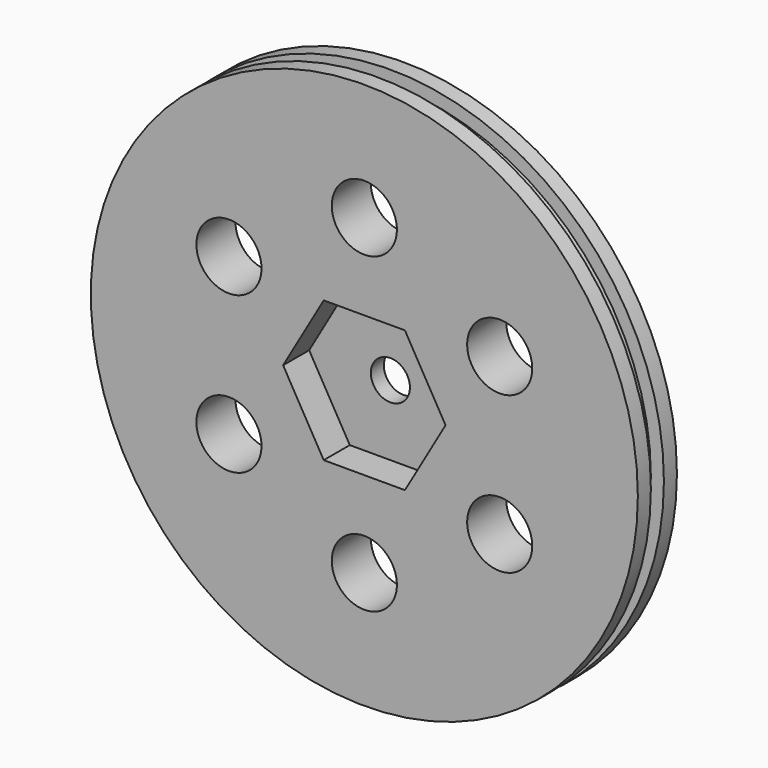
from build123d import *

# Parameters (mm, degrees)
F0_R     = 26.67
F0_R_2   = 25.4
F1_DEPTH = 1.5875
F2_R     = 25.4
F3_DEPTH = 1.5875
F4_R     = 26.67
F4_R_2   = 25.4
F5_DEPTH = 1.5875
F6_R     = 1.905
F7_DEPTH = 25.4
F9_D     = 6.35


# Not quite as in the source:
# - a length typed as a fraction of an inch, garbled in the dataset ("3 / 203.2 mm" for 3/8 in), is restored


with BuildPart() as f1:
    # F0 (on Front) → F1 (new body)
    with BuildSketch(Plane.XZ):
        Circle(F0_R)
        Circle(F0_R_2, mode=Mode.SUBTRACT)
        Circle(F0_R_2)
        with BuildLine():
            ThreePointArc((3.9594681461, 6.858), (6.858, 3.9594681461), (7.9189362922, 0))
            ThreePointArc((7.9189362922, 0), (6.858, -3.9594681461), (3.9594681461, -6.858))
            ThreePointArc((3.9594681461, -6.858), (0, -7.9189362922), (-3.9594681461, -6.858))
            ThreePointArc((-3.9594681461, -6.858), (-6.858, -3.9594681461), (-7.9189362922, 0))
            ThreePointArc((-7.9189362922, 0), (-6.858, 3.9594681461), (-3.9594681461, 6.858))
            ThreePointArc((-3.9594681461, 6.858), (0, 7.9189362922), (3.9594681461, 6.858))
        make_face(mode=Mode.SUBTRACT)
        Polygon((3.9594681461, -6.858), (7.9189362922, 0), (3.9594681461, 6.858), (-3.9594681461, 6.858), (-7.9189362922, 0), (-3.9594681461, -6.858), align=None)
        with BuildLine():
            Line((-3.9594681461, 6.858), (3.9594681461, 6.858))
            ThreePointArc((3.9594681461, 6.858), (0, 7.9189362922), (-3.9594681461, 6.858))
        make_face()
        with BuildLine():
            Line((3.9594681461, 6.858), (7.9189362922, 0))
            ThreePointArc((7.9189362922, 0), (6.858, 3.9594681461), (3.9594681461, 6.858))
        make_face()
        with BuildLine():
            ThreePointArc((3.9594681461, -6.858), (6.858, -3.9594681461), (7.9189362922, 0))
            Line((7.9189362922, 0), (3.9594681461, -6.858))
        make_face()
        with BuildLine():
            ThreePointArc((-3.9594681461, -6.858), (0, -7.9189362922), (3.9594681461, -6.858))
            Line((3.9594681461, -6.858), (-3.9594681461, -6.858))
        make_face()
        with BuildLine():
            ThreePointArc((-7.9189362922, 0), (-6.858, -3.9594681461), (-3.9594681461, -6.858))
            Line((-3.9594681461, -6.858), (-7.9189362922, 0))
        make_face()
        with BuildLine():
            Line((-7.9189362922, 0), (-3.9594681461, 6.858))
            ThreePointArc((-3.9594681461, 6.858), (-6.858, 3.9594681461), (-7.9189362922, 0))
        make_face()
    extrude(amount=F1_DEPTH)

    # F2 (on face) → F3 (join)
    with BuildSketch(Plane.XZ.offset(1.5875)):
        Circle(F2_R)
        with BuildLine():
            ThreePointArc((3.9594681461, 6.858), (6.858, 3.9594681461), (7.9189362922, 0))
            ThreePointArc((7.9189362922, 0), (6.858, -3.9594681461), (3.9594681461, -6.858))
            ThreePointArc((3.9594681461, -6.858), (0, -7.9189362922), (-3.9594681461, -6.858))
            ThreePointArc((-3.9594681461, -6.858), (-6.858, -3.9594681461), (-7.9189362922, 0))
            ThreePointArc((-7.9189362922, 0), (-6.858, 3.9594681461), (-3.9594681461, 6.858))
            ThreePointArc((-3.9594681461, 6.858), (0, 7.9189362922), (3.9594681461, 6.858))
        make_face(mode=Mode.SUBTRACT)
        with BuildLine():
            Line((3.9594681461, 6.858), (7.9189362922, 0))
            ThreePointArc((7.9189362922, 0), (6.858, 3.9594681461), (3.9594681461, 6.858))
        make_face()
        with BuildLine():
            Line((-3.9594681461, 6.858), (3.9594681461, 6.858))
            ThreePointArc((3.9594681461, 6.858), (0, 7.9189362922), (-3.9594681461, 6.858))
        make_face()
        with BuildLine():
            Line((-7.9189362922, 0), (-3.9594681461, 6.858))
            ThreePointArc((-3.9594681461, 6.858), (-6.858, 3.9594681461), (-7.9189362922, 0))
        make_face()
        with BuildLine():
            ThreePointArc((-7.9189362922, 0), (-6.858, -3.9594681461), (-3.9594681461, -6.858))
            Line((-3.9594681461, -6.858), (-7.9189362922, 0))
        make_face()
        with BuildLine():
            ThreePointArc((-3.9594681461, -6.858), (0, -7.9189362922), (3.9594681461, -6.858))
            Line((3.9594681461, -6.858), (-3.9594681461, -6.858))
        make_face()
        with BuildLine():
            ThreePointArc((3.9594681461, -6.858), (6.858, -3.9594681461), (7.9189362922, 0))
            Line((7.9189362922, 0), (3.9594681461, -6.858))
        make_face()
    extrude(amount=F3_DEPTH)

    # F4 (on face) + F0 (on Front) → F5 (join)
    with BuildSketch(Plane.XZ.offset(3.175)):
        Circle(F4_R)
        Circle(F4_R_2, mode=Mode.SUBTRACT)
        Circle(F4_R_2)
        Polygon((7.9189362922, 0), (3.9594681461, -6.858), (-3.9594681461, -6.858), (-7.9189362922, 0), (-3.9594681461, 6.858), (3.9594681461, 6.858), align=None, mode=Mode.SUBTRACT)
    with BuildSketch(Plane.XZ):
        Circle(F0_R)
        Circle(F0_R_2, mode=Mode.SUBTRACT)
    extrude(amount=F5_DEPTH)

    # F6 (on face) → F7 (cut)
    with BuildSketch(Plane.XZ.offset(1.5875)):
        Circle(F6_R)
    extrude(amount=-F7_DEPTH, mode=Mode.SUBTRACT)

    # F9 (through all)
    with Locations(Plane.XZ.offset(4.7625)):
        with Locations((0, 15.24), (0, -15.24), (-13.1982271537, -7.62), (-13.1982271537, 7.62), (13.1982271537, 7.62), (13.1982271537, -7.62)):
            Hole(F9_D / 2)


solid = f1.part
